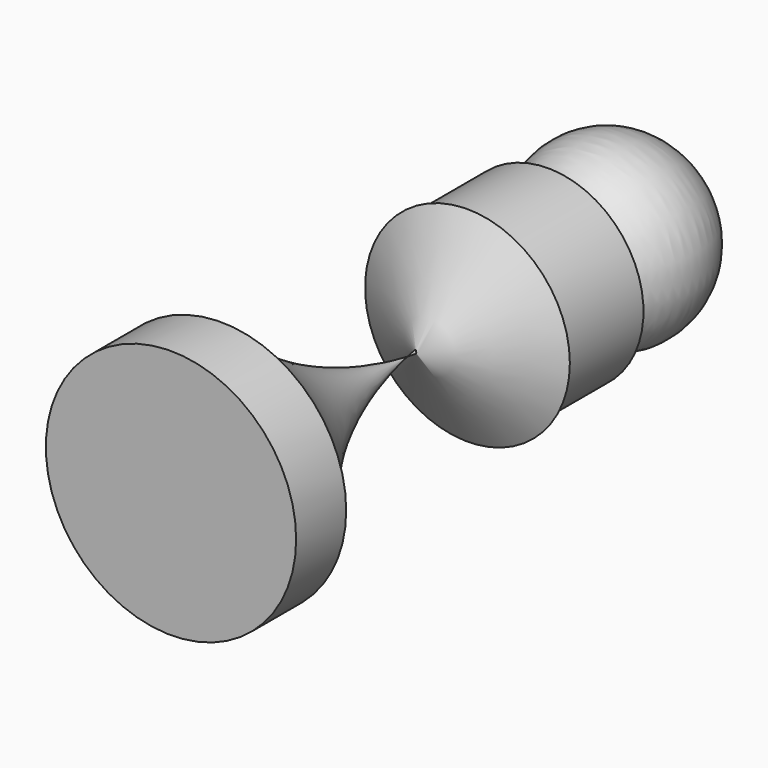
from build123d import *

# Parameters (mm, degrees)
F4_W = 4.8207454383
F4_H = 5.0366010983


with BuildPart() as f1:
    # F0 (on Top) → F1 (revolve)
    with BuildSketch(Plane.XY):
        with BuildLine():
            Line((22.6984173059, -11.7580974475), (22.6984173059, -26.7239958048))
            Line((22.6984173059, -26.7239958048), (29.030142352, -26.7239958048))
            Line((29.030142352, -26.7239958048), (29.030142352, -23.5581323504))
            ThreePointArc((29.030142352, -23.5581323504), (24.8785219503, -18.1870580674), (22.6984173059, -11.7580974475))
        make_face()
    revolve(axis=Axis((22.6984173059, -15.931280097, 0), (0, 1, 0)))


with BuildPart() as f1b:
    # F0 (on Top) → F1, piece 2 (revolve)
    with BuildSketch(Plane.XY):
        with BuildLine():
            ThreePointArc((22.6984173059, -5.1385643892), (22.4307549758, -8.4483309183), (22.6984173059, -11.7580974475))
            Line((22.6984173059, -11.7580974475), (22.6984173059, -5.1385643892))
        make_face()
    revolve(axis=Axis((22.6984173059, -15.931280097, 0), (0, 1, 0)))

    # F2 (on Top) → F3 (revolve)
    with BuildSketch(Plane.XY):
        Polygon((22.8805579245, -8.2024643198), (22.8805579245, -11.3683268428), (28.0610602349, -8.2024643198), align=None)
    revolve(axis=Axis((22.8805579245, -7.4829495279, 0), (0, -1, 0)))

    # F4 (on Top) → F5 (revolve)
    with BuildSketch(Plane.XY):
        with Locations((20.3443262726, -5.4561108118)):
            Rectangle(F4_W, F4_H)
    revolve(axis=Axis((22.7546989918, -5.4561108118, 0), (0, 1, 0)))


with BuildPart() as f1c:
    # F0 (on Top) → F1, piece 3 (revolve)
    with BuildSketch(Plane.XY):
        with BuildLine():
            Line((22.6984173059, 4.9346373416), (22.6984173059, -2.8361182194))
            ThreePointArc((22.6984173059, -2.8361182194), (27.2570955723, 1.0492595611), (22.6984173059, 4.9346373416))
        make_face()
    revolve(axis=Axis((22.6984173059, -15.931280097, 0), (0, 1, 0)))


solid = Compound([f1.part, f1b.part, f1c.part])
